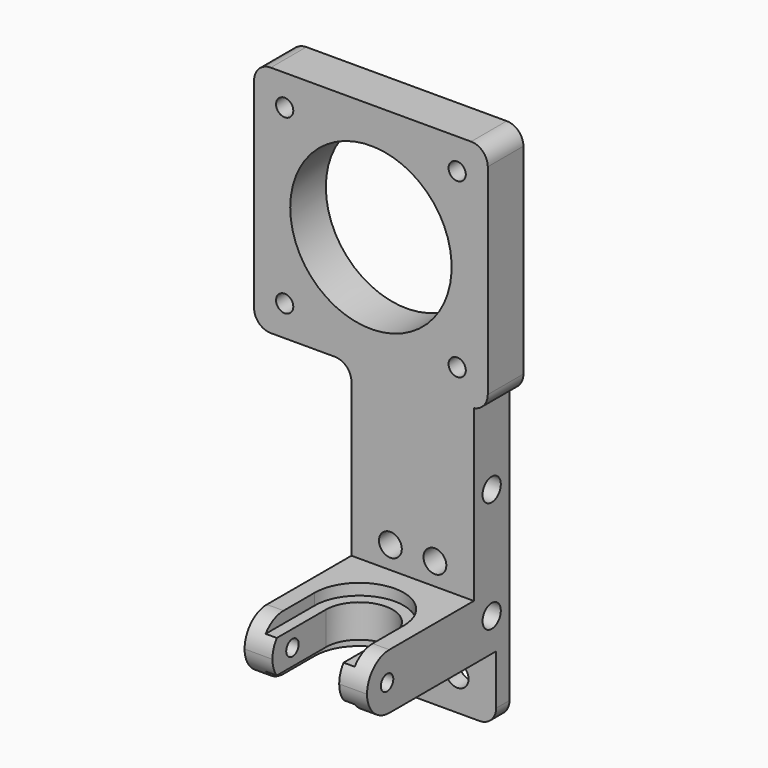
from build123d import *

# Parameters (mm, degrees)
F0_W          = 22
F0_H          = 42
F1_DEPTH      = 3
F2_W          = 3
F2_H          = 30
F2_W_2        = 5
F3_DEPTH      = 22
F4_D          = 4.1
F7_DEPTH      = 5
F8_DEPTH      = 2.97
F9_R          = 4.99999
F11_D         = 4.1
F12_D         = 2.8
F13_W         = 22
F13_H         = 10.5
F14_DEPTH     = 8
F15_T1_DEPTH  = 8
F15_T3_DEPTH  = 18
F15_T5_DEPTH  = 18
F15_T7_DEPTH  = 22.7901994578
F15_T9_DEPTH  = 23
F15_T11_DEPTH = 23
F15_T13_DEPTH = 23
F16_D         = 29
F17_D         = 3.1


# Not quite as in the source:
# - a fillet or chamfer that OpenCascade refuses, or shapes differently, is made with other operations: its cross-section is extruded or revolved along the edge and cut away or added
# - a fillet or chamfer is up to 0.001 mm smaller than in the source, because OpenCascade refuses the exact size


with BuildPart() as f1:
    # F0 (on Front) → F1 (new body)
    with BuildSketch(Plane.XZ):
        with Locations((-28.9233987555, 27.9422005266)):
            Rectangle(F0_W, F0_H)
    extrude(amount=F1_DEPTH)

    # F2 (on face) → F3 (join)
    with BuildSketch(Plane(origin=(-39.9233987555, 0, 0), x_dir=(0, -1, 0), z_dir=(-1, 0, 0))):
        with Locations((1.5, 33.9422005266)):
            Rectangle(F2_W, F2_H)
        with Locations((5.5, 33.9422005266)):
            Rectangle(F2_W_2, F2_H)
    extrude(amount=-F3_DEPTH)

    # F4 (through all)
    with Locations(Plane(origin=(0, 0, 0), x_dir=(1, 0, 0), z_dir=(0, 1, 0))):
        with Locations((-24.9233987555, -12.9422005266), (-32.9233987555, -12.9422005266), (-32.9233987555, -32.9422005266), (-24.9233987555, -32.9422005266)):
            Hole(F4_D / 2)

    # F6 (on line) → F7 (join, symmetric)
    with BuildSketch(Plane.XY.offset(23.9422005266)):
        with BuildLine():
            ThreePointArc((-36.9233987555, -20), (-28.9233987555, -12), (-20.9233987555, -20))
            Line((-20.9233987555, -20), (-20.9233987555, -32))
            Line((-20.9233987555, -32), (-17.9233987555, -32))
            Line((-17.9233987555, -32), (-17.9233987555, 0))
            Line((-17.9233987555, 0), (-39.9233987555, 0))
            Line((-39.9233987555, 0), (-39.9233987555, -32))
            Line((-39.9233987555, -32), (-36.9233987555, -32))
            Line((-36.9233987555, -32), (-36.9233987555, -20))
        make_face()
    extrude(amount=F7_DEPTH, both=True)

    # F6 (on line) → F8 (join, symmetric)
    with BuildSketch(Plane.XY.offset(23.9422005266)):
        with BuildLine():
            ThreePointArc((-34.9233987555, -20), (-28.9233987555, -14), (-22.9233987555, -20))
            Line((-22.9233987555, -20), (-22.9233987555, -25.2915026221))
            ThreePointArc((-22.9233987555, -25.2915026221), (-21.4400839819, -22.8284271247), (-20.9233987555, -20))
            ThreePointArc((-20.9233987555, -20), (-28.9233987555, -12), (-36.9233987555, -20))
            ThreePointArc((-36.9233987555, -20), (-36.406713529, -22.8284271247), (-34.9233987555, -25.2915026221))
            Line((-34.9233987555, -25.2915026221), (-34.9233987555, -20))
        make_face()
        with BuildLine():
            Line((-34.9233987555, -32), (-34.9233987555, -25.2915026221))
            ThreePointArc((-34.9233987555, -25.2915026221), (-36.406713529, -22.8284271247), (-36.9233987555, -20))
            Line((-36.9233987555, -20), (-36.9233987555, -32))
            Line((-36.9233987555, -32), (-34.9233987555, -32))
        make_face()
        with BuildLine():
            ThreePointArc((-20.9233987555, -20), (-21.4400839819, -22.8284271247), (-22.9233987555, -25.2915026221))
            Line((-22.9233987555, -25.2915026221), (-22.9233987555, -32))
            Line((-22.9233987555, -32), (-20.9233987555, -32))
            Line((-20.9233987555, -32), (-20.9233987555, -20))
        make_face()
    extrude(amount=F8_DEPTH, both=True)

    # F9 (radius 5 in the source; OpenCascade refuses exactly that, so slightly less here)
    f9_edges = [f1.edges().sort_by_distance(p)[0] for p in [
        (-38.423399, -32, 28.942201),
        (-38.423399, -32, 18.942201),
        (-19.423399, -32, 18.942201),
        (-19.423399, -32, 28.942201),
    ]]
    fillet(f9_edges, radius=F9_R)

    # F11 (through all)
    with Locations(Plane(origin=(-39.9233987555, 0, 0), x_dir=(0, -1, 0), z_dir=(-1, 0, 0))):
        with Locations((4, 44.9422005266), (4, 24.9422005266)):
            Hole(F11_D / 2)

    # F12 (through all)
    with Locations(Plane(origin=(-39.9233987555, 0, 0), x_dir=(0, -1, 0), z_dir=(-1, 0, 0))):
        with Locations((27.5, 23.9422005266)):
            Hole(F12_D / 2)

    # F13 (on Front) → F14 (join)
    with BuildSketch(Plane.XZ):
        Polygon((-57.4233987555, 59.4422005266), (-39.9233987555, 59.4422005266), (-17.9233987555, 59.4422005266), (-15.4233987555, 59.4422005266), (-15.4233987555, 101.4422005266), (-57.4233987555, 101.4422005266), align=None)
        with Locations((-28.9233987555, 54.1922005266)):
            Rectangle(F13_W, F13_H)
    extrude(amount=F14_DEPTH)

    # F15: fillet of radius 3 on 7 edges, made by hand

    # F15_s2 → F15_t1 (join)
    with BuildSketch(Plane.XZ):
        with BuildLine():
            ThreePointArc((-39.9233987555, 56.4422005266), (-40.8020784119, 58.5635208702), (-42.9233987555, 59.4422005266))
            Line((-42.9233987555, 59.4422005266), (-39.9233987555, 59.4422005266))
            Line((-39.9233987555, 59.4422005266), (-39.9233987555, 56.4422005266))
        make_face()
    extrude(amount=F15_T1_DEPTH)

    # F15_s4 → F15_t3 (cut)
    with BuildSketch(Plane.XZ.offset(-7.5)):
        with BuildLine():
            ThreePointArc((-39.9233987555, 9.9422005266), (-39.0447190991, 7.820880183), (-36.9233987555, 6.9422005266))
            Line((-36.9233987555, 6.9422005266), (-39.9233987555, 6.9422005266))
            Line((-39.9233987555, 6.9422005266), (-39.9233987555, 9.9422005266))
        make_face()
    extrude(amount=F15_T3_DEPTH, mode=Mode.SUBTRACT)

    # F15_s6 → F15_t5 (cut)
    with BuildSketch(Plane.XZ.offset(-7.5)):
        with BuildLine():
            ThreePointArc((-17.9233987555, 9.9422005266), (-18.8020784119, 7.820880183), (-20.9233987555, 6.9422005266))
            Line((-20.9233987555, 6.9422005266), (-17.9233987555, 6.9422005266))
            Line((-17.9233987555, 6.9422005266), (-17.9233987555, 9.9422005266))
        make_face()
    extrude(amount=F15_T5_DEPTH, mode=Mode.SUBTRACT)

    # F15_s8 → F15_t7 (cut)
    with BuildSketch(Plane.XZ.offset(-7.3950997289)):
        with BuildLine():
            ThreePointArc((-17.9233987555, 59.4422005266), (-16.132110908, 60.463748745), (-15.4233987555, 62.4002404181))
            Line((-15.4233987555, 62.4002404181), (-15.4233987555, 59.4422005266))
            Line((-15.4233987555, 59.4422005266), (-17.9233987555, 59.4422005266))
        make_face()
    extrude(amount=F15_T7_DEPTH, mode=Mode.SUBTRACT)

    # F15_s10 → F15_t9 (cut)
    with BuildSketch(Plane.XZ.offset(-7.5)):
        with BuildLine():
            ThreePointArc((-18.4233987555, 101.4422005266), (-16.3020784119, 100.5635208702), (-15.4233987555, 98.4422005266))
            Line((-15.4233987555, 98.4422005266), (-15.4233987555, 101.4422005266))
            Line((-15.4233987555, 101.4422005266), (-18.4233987555, 101.4422005266))
        make_face()
    extrude(amount=F15_T9_DEPTH, mode=Mode.SUBTRACT)

    # F15_s12 → F15_t11 (cut)
    with BuildSketch(Plane.XZ.offset(-7.5)):
        with BuildLine():
            ThreePointArc((-57.4233987555, 98.4422005266), (-56.5447190991, 100.5635208702), (-54.4233987555, 101.4422005266))
            Line((-54.4233987555, 101.4422005266), (-57.4233987555, 101.4422005266))
            Line((-57.4233987555, 101.4422005266), (-57.4233987555, 98.4422005266))
        make_face()
    extrude(amount=F15_T11_DEPTH, mode=Mode.SUBTRACT)

    # F15_s14 → F15_t13 (cut)
    with BuildSketch(Plane.XZ.offset(-7.5)):
        with BuildLine():
            ThreePointArc((-54.4233987555, 59.4422005266), (-56.5447190991, 60.320880183), (-57.4233987555, 62.4422005266))
            Line((-57.4233987555, 62.4422005266), (-57.4233987555, 59.4422005266))
            Line((-57.4233987555, 59.4422005266), (-54.4233987555, 59.4422005266))
        make_face()
    extrude(amount=F15_T13_DEPTH, mode=Mode.SUBTRACT)

    # F16 (through all)
    with Locations(Plane(origin=(0, 0, 0), x_dir=(1, 0, 0), z_dir=(0, 1, 0))):
        with Locations((-36.4233987555, -80.4422005266)):
            Hole(F16_D / 2)

    # F17 (through all)
    with Locations(Plane(origin=(0, 0, 0), x_dir=(1, 0, 0), z_dir=(0, 1, 0))):
        with Locations((-51.9233987555, -95.9422005266), (-20.9233987555, -95.9422005266), (-20.9233987555, -64.9422005266), (-51.9233987555, -64.9422005266)):
            Hole(F17_D / 2)


solid = f1.part
